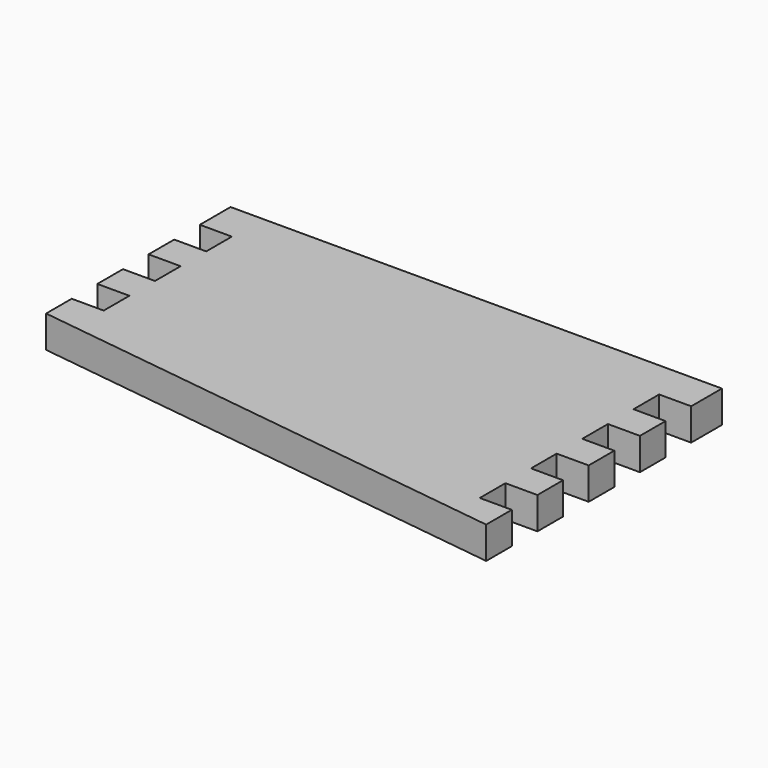
from build123d import *

# Parameters (mm, degrees)
F0_W     = 10
F0_H     = 10
F1_DEPTH = 10


# Not quite as in the source:
# - a feature names something its author has since deleted; it is built from what else it names


with BuildPart() as f1:
    # F0 (on Top) → F1 (new body)
    with BuildSketch(Plane.XY):
        Polygon((-2.2346749902, 36.9413525529), (-135.6346749902, 36.9413525529), (-135.6346749902, 26.9413525529), (-135.6346749902, 16.9413525529), (-135.6346749902, 6.9413525529), (-135.6346749902, -3.0586474471), (-135.6346749902, -13.0586474471), (-135.6346749902, -23.0586474471), (-135.6346749902, -33.0586474471), (-2.2346749902, -33.0586474471), (-2.2346749902, -23.0586474471), (-2.2346749902, -13.0586474471), (-2.2346749902, -3.0586474471), (-2.2346749902, 6.9413525529), (-2.2346749902, 16.9413525529), (-2.2346749902, 26.9413525529), align=None)
        with Locations((-140.6346749902, 31.9413525529)):
            Rectangle(F0_W, F0_H)
        with Locations((-140.6346749902, 11.9413525529)):
            Rectangle(F0_W, F0_H)
        with Locations((-140.6346749902, -8.0586474471)):
            Rectangle(F0_W, F0_H)
        with Locations((-140.6346749902, -28.0586474471)):
            Rectangle(F0_W, F0_H)
        with Locations((2.7653250098, 31.9413525529)):
            Rectangle(F0_W, F0_H)
        with Locations((2.7653250098, 11.9413525529)):
            Rectangle(F0_W, F0_H)
        with Locations((2.7653250098, -8.0586474471)):
            Rectangle(F0_W, F0_H)
        with Locations((2.7653250098, -28.0586474471)):
            Rectangle(F0_W, F0_H)
        Polygon((-135.6346749902, -33.0586474471), (-145.6346749902, -33.0586474471), (-2.2346749902, -51.7548664823), (-2.2346749902, -43.0586474471), (-2.2346749902, -33.0586474471), align=None)
        Polygon((-2.2346749902, -43.0586474471), (-2.2346749902, -51.7548664823), (7.7653250098, -53.0586474471), (7.7653250098, -43.0586474471), align=None)
        Polygon((-145.6346749902, 38.9413525529), (-145.6346749902, 36.9413525529), (-135.6346749902, 36.9413525529), (-2.2346749902, 36.9413525529), (7.7653250098, 36.9413525529), (7.7653250098, 38.9413525529), align=None)
    extrude(amount=F1_DEPTH)


solid = f1.part
